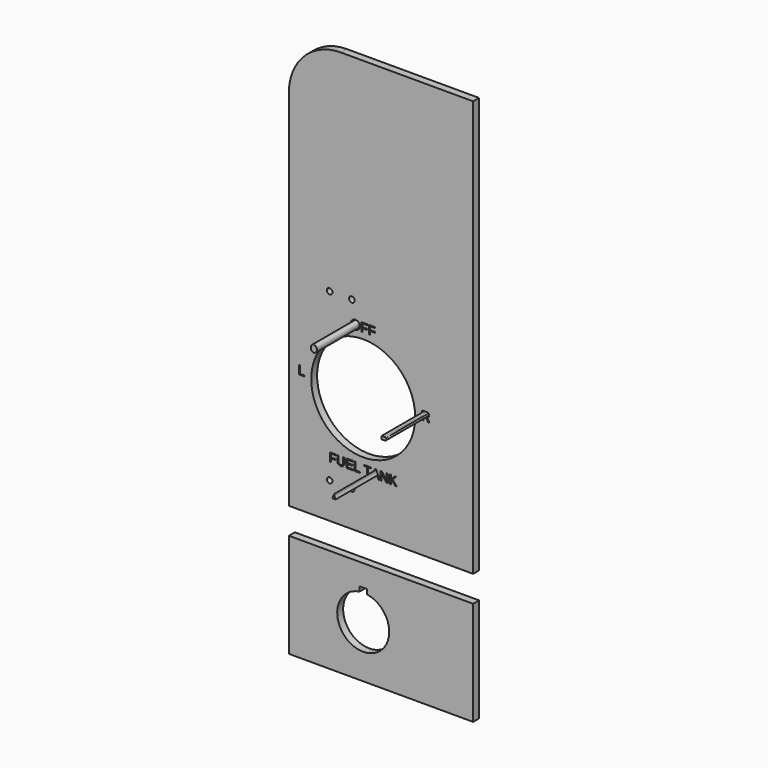
from build123d import *

# Parameters (mm, degrees)
F0_R     = 22.225
F1_DEPTH = 3.175
F2_D     = 2.413
F3_DEPTH = 25.4
F0_W     = 78.74
F0_H     = 44.45
F4_DEPTH = 3.175


with BuildPart() as f1:
    # F0 (on Front) → F1 (new body)
    with BuildSketch(Plane.XZ):
        with BuildLine():
            Line((-78.74, 155.575), (-78.74, 0))
            Line((-78.74, 0), (0, 0))
            Line((0, 0), (0, 177.8))
            Line((0, 177.8), (-56.515, 177.8))
            ThreePointArc((-56.515, 177.8), (-72.2304482119, 171.2904482119), (-78.74, 155.575))
        make_face()
        Polygon((-58.67796875, 25.4628385417), (-60.7706575521, 25.4628385417), (-60.7706575521, 24.1085026042), (-58.7399804687, 24.1085026042), (-58.7399804687, 23.7000520833), (-60.7706575521, 23.7000520833), (-60.7706575521, 22.225), (-61.2642708333, 22.225), (-61.2642708333, 25.8655013021), (-58.67796875, 25.8655013021), align=None, mode=Mode.SUBTRACT)
        Polygon((-72.122109375, 50.8), (-74.4554036458, 50.8), (-74.4554036458, 54.4405013021), (-73.9617903646, 54.4405013021), (-73.9617903646, 51.2034895833), (-72.122109375, 51.2034895833), align=None, mode=Mode.SUBTRACT)
        with BuildLine():
            add(Edge.make_bspline(
                [(-55.7700325521, 22.3424088542), (-56.1123372396, 22.1729101563), (-56.5778385417, 22.1729101563)],
                knots=[0, 0, 0, 1, 1, 1], degree=2))
            add(Edge.make_bspline(
                [(-56.5778385417, 22.1729101563), (-57.0243229167, 22.1729101563), (-57.3575325521, 22.3357942708)],
                knots=[0, 0, 0, 1, 1, 1], degree=2))
            add(Edge.make_bspline(
                [(-57.3575325521, 22.3357942708), (-57.6907421875, 22.4986783854), (-57.874296875, 22.8087369792)],
                knots=[0, 0, 0, 1, 1, 1], degree=2))
            add(Edge.make_bspline(
                [(-57.874296875, 22.8087369792), (-58.0578515625, 23.1187955729), (-58.0578515625, 23.5479166667)],
                knots=[0, 0, 0, 1, 1, 1], degree=2))
            Line((-58.0578515625, 23.5479166667), (-58.0578515625, 25.8655013021))
            Line((-58.0578515625, 25.8655013021), (-57.5642382812, 25.8655013021))
            Line((-57.5642382812, 25.8655013021), (-57.5642382812, 23.5892578125))
            add(Edge.make_bspline(
                [(-57.5642382812, 23.5892578125), (-57.5642382812, 23.0906835938), (-57.3112304687, 22.8323014323)],
                knots=[0, 0, 0, 1, 1, 1], degree=2))
            add(Edge.make_bspline(
                [(-57.3112304687, 22.8323014323), (-57.0582226562, 22.5739192708), (-56.5803190104, 22.5739192708)],
                knots=[0, 0, 0, 1, 1, 1], degree=2))
            add(Edge.make_bspline(
                [(-56.5803190104, 22.5739192708), (-56.0891861979, 22.5739192708), (-55.8167480469, 22.8413964844)],
                knots=[0, 0, 0, 1, 1, 1], degree=2))
            add(Edge.make_bspline(
                [(-55.8167480469, 22.8413964844), (-55.5443098958, 23.1088736979), (-55.5443098958, 23.6231575521)],
                knots=[0, 0, 0, 1, 1, 1], degree=2))
            Line((-55.5443098958, 23.6231575521), (-55.5443098958, 25.8655013021))
            Line((-55.5443098958, 25.8655013021), (-55.0531770833, 25.8655013021))
            Line((-55.0531770833, 25.8655013021), (-55.0531770833, 23.59421875))
            add(Edge.make_bspline(
                [(-55.0531770833, 23.59421875), (-55.0531770833, 23.1526953125), (-55.240452474, 22.8323014323)],
                knots=[0, 0, 0, 1, 1, 1], degree=2))
            add(Edge.make_bspline(
                [(-55.240452474, 22.8323014323), (-55.4277278646, 22.5119075521), (-55.7700325521, 22.3424088542)],
                knots=[0, 0, 0, 1, 1, 1], degree=2))
        make_face(mode=Mode.SUBTRACT)
        Polygon((-51.3423958333, 22.225), (-54.2106445312, 22.225), (-54.2106445312, 25.8655013021), (-51.4482291667, 25.8655013021), (-51.4482291667, 25.4628385417), (-53.71703125, 25.4628385417), (-53.71703125, 24.2945377604), (-51.603671875, 24.2945377604), (-51.603671875, 23.8968359375), (-53.71703125, 23.8968359375), (-53.71703125, 22.6284895833), (-51.3423958333, 22.6284895833), align=None, mode=Mode.SUBTRACT)
        Polygon((-48.3476432292, 22.225), (-50.6809375, 22.225), (-50.6809375, 25.8655013021), (-50.1873242187, 25.8655013021), (-50.1873242187, 22.6284895833), (-48.3476432292, 22.6284895833), align=None, mode=Mode.SUBTRACT)
        Polygon((-43.5909309896, 25.4628385417), (-44.8419140625, 25.4628385417), (-44.8419140625, 22.225), (-45.333046875, 22.225), (-45.333046875, 25.4628385417), (-46.583203125, 25.4628385417), (-46.583203125, 25.8655013021), (-43.5909309896, 25.8655013021), align=None, mode=Mode.SUBTRACT)
        Polygon((-39.9512565104, 22.225), (-40.4547916667, 22.225), (-40.8706835937, 23.2899479167), (-42.5292903646, 23.2899479167), (-42.9484895833, 22.225), (-43.4594661458, 22.225), (-41.9744921875, 25.8655013021), (-41.4130794271, 25.8655013021), align=None, mode=Mode.SUBTRACT)
        with Locations((-46.99, 50.8)):
            Circle(F0_R, mode=Mode.SUBTRACT)
        with BuildLine():
            Line((-36.5505338542, 22.225), (-37.1450195312, 22.225))
            Line((-37.1450195312, 22.225), (-39.0930143229, 25.3255859375))
            Line((-39.0930143229, 25.3255859375), (-39.0797851562, 25.0750585938))
            Line((-39.0797851562, 25.0750585938), (-39.0673828125, 24.6434570313))
            Line((-39.0673828125, 24.6434570313), (-39.0673828125, 22.225))
            Line((-39.0673828125, 22.225), (-39.5064257812, 22.225))
            Line((-39.5064257812, 22.225), (-39.5064257812, 25.8655013021))
            Line((-39.5064257812, 25.8655013021), (-38.9326106771, 25.8655013021))
            Line((-38.9326106771, 25.8655013021), (-36.9639453125, 22.7442447917))
            add(Edge.make_bspline(
                [(-36.9639453125, 22.7442447917), (-36.9945377604, 23.2510872396), (-36.9945377604, 23.4784635417)],
                knots=[0, 0, 0, 1, 1, 1], degree=2))
            Line((-36.9945377604, 23.4784635417), (-36.9945377604, 25.8655013021))
            Line((-36.9945377604, 25.8655013021), (-36.5505338542, 25.8655013021))
            Line((-36.5505338542, 25.8655013021), (-36.5505338542, 22.225))
        make_face(mode=Mode.SUBTRACT)
        Polygon((-32.6487565104, 22.225), (-33.2614322917, 22.225), (-34.7158138021, 23.9819986979), (-35.1912369792, 23.6206770833), (-35.1912369792, 22.225), (-35.6848502604, 22.225), (-35.6848502604, 25.8655013021), (-35.1912369792, 25.8655013021), (-35.1912369792, 24.0415299479), (-33.43671875, 25.8655013021), (-32.8554622396, 25.8655013021), (-34.4057552083, 24.2846158854), align=None, mode=Mode.SUBTRACT)
        with BuildLine():
            Line((-18.6489908854, 50.8), (-19.2170182292, 50.8))
            Line((-19.2170182292, 50.8), (-20.1629036458, 52.3114322917))
            Line((-20.1629036458, 52.3114322917), (-21.2973046875, 52.3114322917))
            Line((-21.2973046875, 52.3114322917), (-21.2973046875, 50.8))
            Line((-21.2973046875, 50.8), (-21.7909179687, 50.8))
            Line((-21.7909179687, 50.8), (-21.7909179687, 54.4405013021))
            Line((-21.7909179687, 54.4405013021), (-20.0777408854, 54.4405013021))
            add(Edge.make_bspline(
                [(-20.0777408854, 54.4405013021), (-19.4625846354, 54.4405013021), (-19.1281347656, 54.1655826823)],
                knots=[0, 0, 0, 1, 1, 1], degree=2))
            add(Edge.make_bspline(
                [(-19.1281347656, 54.1655826823), (-18.7936848958, 53.8906640625), (-18.7936848958, 53.39953125)],
                knots=[0, 0, 0, 1, 1, 1], degree=2))
            add(Edge.make_bspline(
                [(-18.7936848958, 53.39953125), (-18.7936848958, 52.9935611979), (-19.03015625, 52.7169889323)],
                knots=[0, 0, 0, 1, 1, 1], degree=2))
            add(Edge.make_bspline(
                [(-19.03015625, 52.7169889323), (-19.2666276042, 52.4404166667), (-19.6825195312, 52.3684830729)],
                knots=[0, 0, 0, 1, 1, 1], degree=2))
            Line((-19.6825195312, 52.3684830729), (-18.6489908854, 50.8))
        make_face(mode=Mode.SUBTRACT)
        with BuildLine():
            add(Edge.make_bspline(
                [(-48.7106184896, 78.3968684896), (-48.4948177083, 77.976015625), (-48.4948177083, 77.4022005208)],
                knots=[0, 0, 0, 1, 1, 1], degree=2))
            add(Edge.make_bspline(
                [(-48.4948177083, 77.4022005208), (-48.4948177083, 76.8308658854), (-48.7130989583, 76.4021582031)],
                knots=[0, 0, 0, 1, 1, 1], degree=2))
            add(Edge.make_bspline(
                [(-48.7130989583, 76.4021582031), (-48.9313802083, 75.9734505208), (-49.3398307292, 75.7431803385)],
                knots=[0, 0, 0, 1, 1, 1], degree=2))
            add(Edge.make_bspline(
                [(-49.3398307292, 75.7431803385), (-49.74828125, 75.5129101563), (-50.30390625, 75.5129101563)],
                knots=[0, 0, 0, 1, 1, 1], degree=2))
            add(Edge.make_bspline(
                [(-50.30390625, 75.5129101563), (-50.8644921875, 75.5129101563), (-51.2712890625, 75.7406998698)],
                knots=[0, 0, 0, 1, 1, 1], degree=2))
            add(Edge.make_bspline(
                [(-51.2712890625, 75.7406998698), (-51.6780859375, 75.9684895833), (-51.8926464844, 76.3984375)],
                knots=[0, 0, 0, 1, 1, 1], degree=2))
            add(Edge.make_bspline(
                [(-51.8926464844, 76.3984375), (-52.1072070312, 76.8283854167), (-52.1072070312, 77.4022005208)],
                knots=[0, 0, 0, 1, 1, 1], degree=2))
            add(Edge.make_bspline(
                [(-52.1072070312, 77.4022005208), (-52.1072070312, 78.2753255208), (-51.6293033854, 78.7676985677)],
                knots=[0, 0, 0, 1, 1, 1], degree=2))
            add(Edge.make_bspline(
                [(-51.6293033854, 78.7676985677), (-51.1513997396, 79.2600716146), (-50.2981184896, 79.2600716146)],
                knots=[0, 0, 0, 1, 1, 1], degree=2))
            add(Edge.make_bspline(
                [(-50.2981184896, 79.2600716146), (-49.7424934896, 79.2600716146), (-49.3344563802, 79.0388964844)],
                knots=[0, 0, 0, 1, 1, 1], degree=2))
            add(Edge.make_bspline(
                [(-49.3344563802, 79.0388964844), (-48.9264192708, 78.8177213542), (-48.7106184896, 78.3968684896)],
                knots=[0, 0, 0, 1, 1, 1], degree=2))
        make_face(mode=Mode.SUBTRACT)
        Polygon((-45.2214257812, 78.8028385417), (-47.3141145833, 78.8028385417), (-47.3141145833, 77.4485026042), (-45.2834375, 77.4485026042), (-45.2834375, 77.0400520833), (-47.3141145833, 77.0400520833), (-47.3141145833, 75.565), (-47.8077278646, 75.565), (-47.8077278646, 79.2055013021), (-45.2214257812, 79.2055013021), align=None, mode=Mode.SUBTRACT)
        Polygon((-41.989375, 78.8028385417), (-44.0820638021, 78.8028385417), (-44.0820638021, 77.4485026042), (-42.0513867188, 77.4485026042), (-42.0513867188, 77.0400520833), (-44.0820638021, 77.0400520833), (-44.0820638021, 75.565), (-44.5756770833, 75.565), (-44.5756770833, 79.2055013021), (-41.989375, 79.2055013021), align=None, mode=Mode.SUBTRACT)
    extrude(amount=F1_DEPTH)

    # F2 (through all)
    with Locations(Plane(origin=(0, 0, 0), x_dir=(1, 0, 0), z_dir=(0, 1, 0))):
        with Locations((-51.816, -86.36), (-61.341, -86.36), (-61.341, -15.24), (-51.816, -15.24)):
            Hole(F2_D / 2)


with BuildPart() as f3:
    # F0 (on Front) → F3 (new body)
    with BuildSketch(Plane.XZ):
        with BuildLine():
            add(Edge.make_bspline(
                [(-49.3356966146, 76.3029394531), (-48.9983528646, 76.6919596354), (-48.9983528646, 77.4022005208)],
                knots=[0, 0, 0, 1, 1, 1], degree=2))
            add(Edge.make_bspline(
                [(-48.9983528646, 77.4022005208), (-48.9983528646, 78.0818489583), (-49.3381770833, 78.4692154948)],
                knots=[0, 0, 0, 1, 1, 1], degree=2))
            add(Edge.make_bspline(
                [(-49.3381770833, 78.4692154948), (-49.6780013021, 78.8565820313), (-50.2981184896, 78.8565820313)],
                knots=[0, 0, 0, 1, 1, 1], degree=2))
            add(Edge.make_bspline(
                [(-50.2981184896, 78.8565820313), (-50.9240234375, 78.8565820313), (-51.2650878906, 78.4741764323)],
                knots=[0, 0, 0, 1, 1, 1], degree=2))
            add(Edge.make_bspline(
                [(-51.2650878906, 78.4741764323), (-51.6061523437, 78.0917708333), (-51.6061523437, 77.4022005208)],
                knots=[0, 0, 0, 1, 1, 1], degree=2))
            add(Edge.make_bspline(
                [(-51.6061523437, 77.4022005208), (-51.6061523437, 76.7175911458), (-51.260953776, 76.3157552083)],
                knots=[0, 0, 0, 1, 1, 1], degree=2))
            add(Edge.make_bspline(
                [(-51.260953776, 76.3157552083), (-50.9157552083, 75.9139192708), (-50.30390625, 75.9139192708)],
                knots=[0, 0, 0, 1, 1, 1], degree=2))
            add(Edge.make_bspline(
                [(-50.30390625, 75.9139192708), (-49.6730403646, 75.9139192708), (-49.3356966146, 76.3029394531)],
                knots=[0, 0, 0, 1, 1, 1], degree=2))
        make_face()
    extrude(amount=F3_DEPTH)


with BuildPart() as f3b:
    # F0 (on Front) → F3, piece 2 (new body)
    with BuildSketch(Plane.XZ):
        with BuildLine():
            add(Edge.make_bspline(
                [(-19.5030989583, 52.8840071615), (-19.2897786458, 53.0663216146), (-19.2897786458, 53.3945703125)],
                knots=[0, 0, 0, 1, 1, 1], degree=2))
            add(Edge.make_bspline(
                [(-19.2897786458, 53.3945703125), (-19.2897786458, 53.7120703125), (-19.5055794271, 53.8786751302)],
                knots=[0, 0, 0, 1, 1, 1], degree=2))
            add(Edge.make_bspline(
                [(-19.5055794271, 53.8786751302), (-19.7213802083, 54.0452799479), (-20.1265234375, 54.0452799479)],
                knots=[0, 0, 0, 1, 1, 1], degree=2))
            Line((-20.1265234375, 54.0452799479), (-21.2973046875, 54.0452799479))
            Line((-21.2973046875, 54.0452799479), (-21.2973046875, 52.7016927083))
            Line((-21.2973046875, 52.7016927083), (-20.1058528646, 52.7016927083))
            add(Edge.make_bspline(
                [(-20.1058528646, 52.7016927083), (-19.7164192708, 52.7016927083), (-19.5030989583, 52.8840071615)],
                knots=[0, 0, 0, 1, 1, 1], degree=2))
        make_face()
    extrude(amount=F3_DEPTH)


with BuildPart() as f3c:
    # F0 (on Front) → F3, piece 3 (new body)
    with BuildSketch(Plane.XZ):
        with BuildLine():
            Line((-41.6305338542, 25.2792838542), (-41.6999869792, 25.4934309896))
            Line((-41.6999869792, 25.4934309896), (-41.7231380208, 25.4214973958))
            add(Edge.make_bspline(
                [(-41.7231380208, 25.4214973958), (-41.7884570312, 25.2065234375), (-41.9149609375, 24.8708333333)],
                knots=[0, 0, 0, 1, 1, 1], degree=2))
            Line((-41.9149609375, 24.8708333333), (-42.3796354167, 23.6744205729))
            Line((-42.3796354167, 23.6744205729), (-41.0178580729, 23.6744205729))
            Line((-41.0178580729, 23.6744205729), (-41.4858398437, 24.8757942708))
            add(Edge.make_bspline(
                [(-41.4858398437, 24.8757942708), (-41.5577734375, 25.0543880208), (-41.6305338542, 25.2792838542)],
                knots=[0, 0, 0, 1, 1, 1], degree=2))
        make_face()
    extrude(amount=F3_DEPTH)


with BuildPart() as f4:
    # F0 (on Front) → F4 (new body)
    with BuildSketch(Plane.XZ):
        with Locations((-39.37, -33.4787629724)):
            Rectangle(F0_W, F0_H)
        with BuildLine():
            ThreePointArc((-45.4025, -22.4802403443), (-46.99, -44.5912629724), (-48.5775, -22.4802403443))
            Line((-48.5775, -22.4802403443), (-48.5775, -20.4482403443))
            Line((-48.5775, -20.4482403443), (-45.4025, -20.4482403443))
            Line((-45.4025, -20.4482403443), (-45.4025, -22.4802403443))
        make_face(mode=Mode.SUBTRACT)
    extrude(amount=F4_DEPTH)


solid = Compound([f1.part, f3.part, f3b.part, f3c.part, f4.part])
